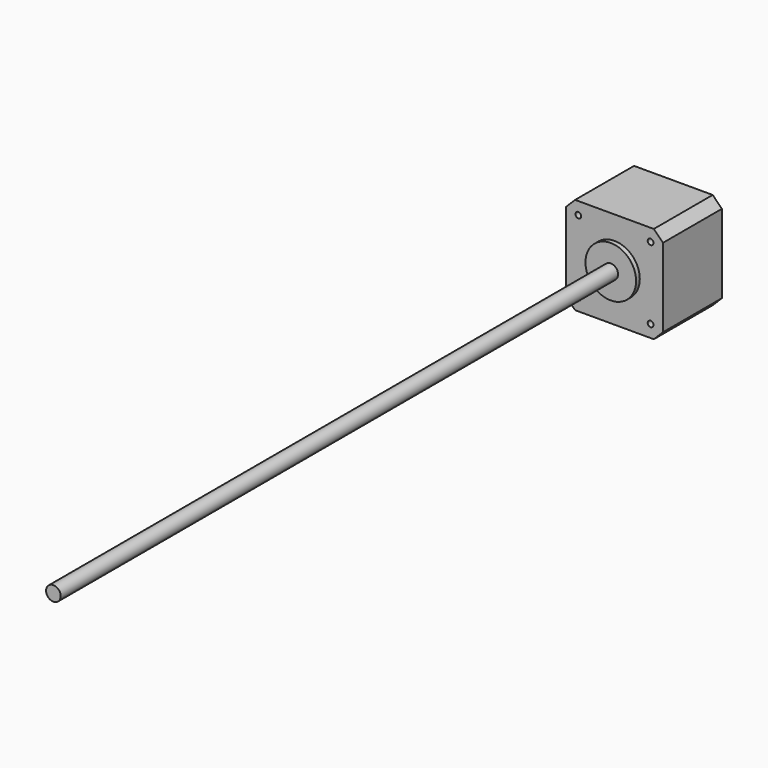
from build123d import *

# Parameters (mm, degrees)
F0_W     = 42.2
F0_H     = 42.2
F0_R     = 1.25
F0_R_2   = 11
F0_R_3   = 3.175
F1_DEPTH = 32
F2_DEPTH = 304.8
F3_DEPTH = 2
F4_DEPTH = 3.8
F5_SIZE  = 4


with BuildPart() as f1:
    # F0 (on Front) → F1 (new body)
    with BuildSketch(Plane.XZ):
        Rectangle(F0_W, F0_H)
        with Locations((-15.7, -15.7)):
            Circle(F0_R, mode=Mode.SUBTRACT)
        with Locations((15.7, -15.7)):
            Circle(F0_R, mode=Mode.SUBTRACT)
        with Locations((-15.7, 15.7)):
            Circle(F0_R, mode=Mode.SUBTRACT)
        Circle(F0_R_2, mode=Mode.SUBTRACT)
        with Locations((15.7, 15.7)):
            Circle(F0_R, mode=Mode.SUBTRACT)
        with Locations((15.7, 15.7)):
            Circle(F0_R)
        with Locations((15.7, -15.7)):
            Circle(F0_R)
        with Locations((-15.7, -15.7)):
            Circle(F0_R)
        with Locations((-15.7, 15.7)):
            Circle(F0_R)
        Circle(F0_R_2)
        Circle(F0_R_3, mode=Mode.SUBTRACT)
        Circle(F0_R_3)
    extrude(amount=-F1_DEPTH)

    # F0 (on Front) → F3 (join)
    with BuildSketch(Plane.XZ):
        Circle(F0_R_2)
        Circle(F0_R_3, mode=Mode.SUBTRACT)
    extrude(amount=F3_DEPTH)

    # F0 (on Front) → F4 (cut)
    with BuildSketch(Plane.XZ):
        with Locations((-15.7, 15.7)):
            Circle(F0_R)
        with Locations((15.7, 15.7)):
            Circle(F0_R)
        with Locations((15.7, -15.7)):
            Circle(F0_R)
        with Locations((-15.7, -15.7)):
            Circle(F0_R)
    extrude(amount=-F4_DEPTH, mode=Mode.SUBTRACT)

    # F5
    f5_edges = [f1.edges().sort_by_distance(p)[0] for p in [
        (-21.1, 16, 21.1),
        (21.1, 16, 21.1),
        (21.1, 16, -21.1),
        (-21.1, 16, -21.1),
    ]]
    chamfer(f5_edges, length=F5_SIZE)


with BuildPart() as f2:
    # F0 (on Front) → F2 (new body)
    with BuildSketch(Plane.XZ):
        Circle(F0_R_3)
    extrude(amount=F2_DEPTH)


solid = Compound([f1.part, f2.part])
